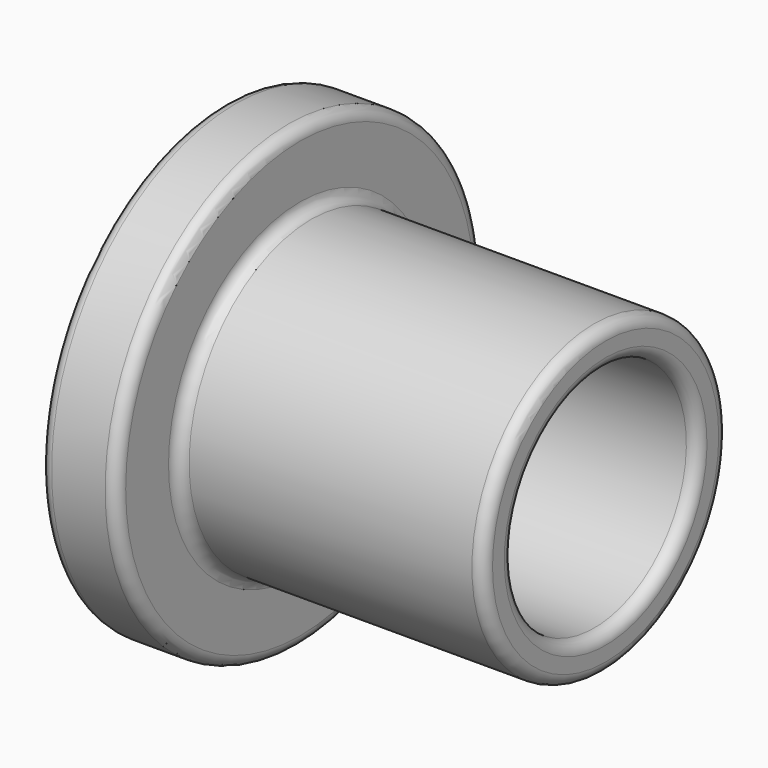
from build123d import *

# Parameters (mm, degrees)
F5_R = 3
F6_R = 5.08


# Not quite as in the source:
# - a feature of the source that left no trace in its solid (it failed there, or was rolled back) is left out
# - the program builds the solid bodies; features that only make, move or delete a surface that nothing else refers to are left out


with BuildPart() as f4:
    # F3 (on Front) → F4 (revolve)
    with BuildSketch(Plane.XZ):
        Polygon((-47.3268434405, -77.5008672476), (-47.3268434405, -127.3418408632), (-27.3268434405, -127.3418408632), (-27.3268434405, -107.3418408632), (52.6731565595, -107.3418408632), (52.6731565595, -97.5008672476), (-27.3268434405, -97.5008672476), (-27.3268434405, -77.5008672476), align=None)
    revolve(axis=Axis((2.6731565595, 0, -137.5008672476), (1, 0, 0)))

    # F5
    f5_edges = [f4.edges().sort_by_distance(p)[0] for p in [
        (52.673157, 0, -167.659894),
        (52.673157, 0, -177.500867),
        (-27.326843, 0, -177.500867),
        (-27.326843, 0, -197.500867),
        (-47.326843, 0, -197.500867),
    ]]
    fillet(f5_edges, radius=F5_R)

    # F6
    f6_edges = [f4.edges().sort_by_distance(p)[0] for p in [
        (-47.326843, 0, -147.659894),
    ]]
    fillet(f6_edges, radius=F6_R)


solid = f4.part
